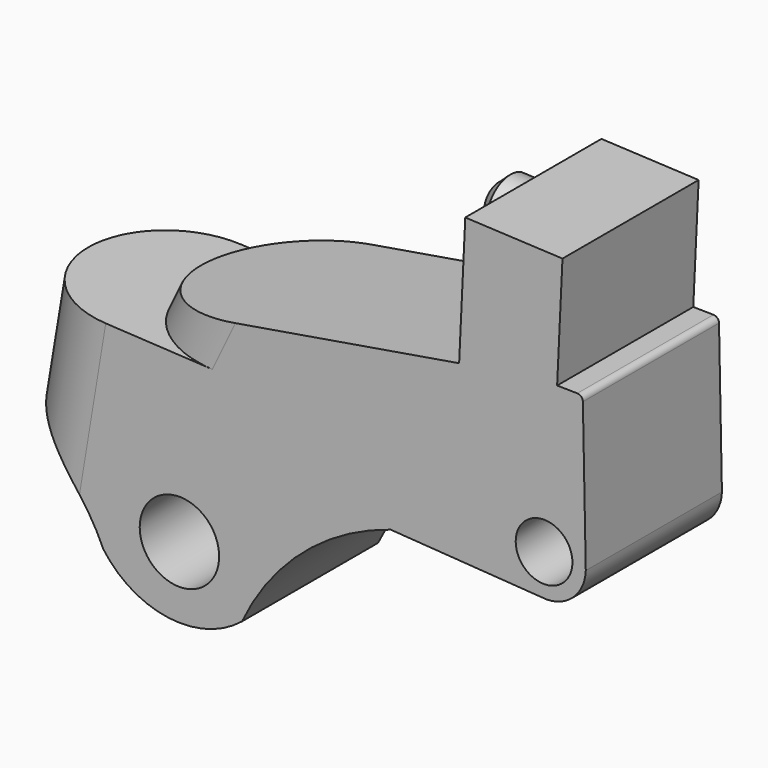
from build123d import *

# Parameters (mm, degrees)
F1_DEPTH = 3.81
F2_D     = 1.778
F3_D     = 1.27
F4_R     = 1.90499
F5_DEPTH = 2.921
F6_R     = 0.636089801
F7_DEPTH = 0.762
F8_SIZE  = 0.254
F9_R     = 0.127


# Not quite as in the source:
# - a fillet or chamfer is up to 0.001 mm smaller than in the source, because OpenCascade refuses the exact size
# - a feature names something its author has since deleted; it is built from what else it names


with BuildPart() as f1:
    # F0 (on Front) → F1 (new body)
    with BuildSketch(Plane.XZ):
        with BuildLine():
            Line((-39.4140869416, 30.484917322), (-39.6941413215, 29.9037330352))
            Line((-39.6941413215, 29.9037330352), (-41.9326054958, 30.025163579))
            Line((-41.9326054958, 30.025163579), (-42.315851897, 27.6998355985))
            ThreePointArc((-42.315851897, 27.6998355985), (-40.9839410359, 26.7856748681), (-40.0724932551, 25.4519060254))
            ThreePointArc((-40.0724932551, 25.4519060254), (-38.6103077884, 24.5752589314), (-36.9695164263, 25.0381845981))
            ThreePointArc((-36.9695164263, 25.0381845981), (-35.6119860231, 26.8367061404), (-33.6415685093, 27.929877378))
            Line((-33.6415685093, 27.929877378), (-30.2701074994, 27.6978733483))
            ThreePointArc((-30.2701074994, 27.6978733483), (-29.5830798604, 27.8997588647), (-29.2723267028, 28.5448923498))
            Line((-29.2723267028, 28.5448923498), (-29.339633882, 31.9740138948))
            Line((-29.339633882, 31.9740138948), (-29.925275594, 31.9827347994))
            Line((-29.925275594, 31.9827347994), (-29.9314986914, 31.6059216857))
            Line((-29.9314986914, 31.6059216857), (-32.1076634707, 31.7085161805))
            Line((-32.1076634707, 31.7085161805), (-39.4140869416, 30.484917322))
        make_face()
    extrude(amount=F1_DEPTH)

    # F2 (through all)
    with Locations(Plane(origin=(0, 0, 0), x_dir=(1, 0, 0), z_dir=(0, 1, 0))):
        with Locations((-38.3695736527, -26.1525325477)):
            Hole(F2_D / 2)

    # F3 (through all)
    with Locations(Plane(origin=(0, 0, 0), x_dir=(1, 0, 0), z_dir=(0, 1, 0))):
        with Locations((-30.2061401308, -28.6094471812)):
            Hole(F3_D / 2)

    # F4 (radius 1.905 in the source; OpenCascade refuses exactly that, so slightly less here)
    f4_edges = [f1.edges().sort_by_distance(p)[0] for p in [
        (-42.124229, -3.81, 28.8625),
        (-42.124229, 0, 28.8625),
        (-39.554114, -3.81, 30.194325),
        (-39.554114, 0, 30.194325),
    ]]
    fillet(f4_edges, radius=F4_R)

    # F5 (add): a face of the model
    f5_faces = [f1.faces().sort_by_distance(p)[0] for p in [
        (-31.0195810811, -1.905, 31.6572189331),
    ]]
    extrude(f5_faces, amount=F5_DEPTH)

    # F6 (on face) → F7 (join)
    with BuildSketch(Plane(origin=(-33.5280299441, 0, 1.5806667432), x_dir=(0, -1, 0), z_dir=(-0.9988905408, 0, 0.0470923302))):
        with Locations((1.905, 32.3275662959)):
            Circle(F6_R)
    extrude(amount=F7_DEPTH)

    # F8
    f8_edges = [f1.edges().sort_by_distance(p)[0] for p in [
        (-32.766804, -1.26891, 33.908251),
    ]]
    chamfer(f8_edges, length=F8_SIZE)

    # F9
    f9_edges = [f1.edges().sort_by_distance(p)[0] for p in [
        (-29.339634, -1.905, 31.974014),
    ]]
    fillet(f9_edges, radius=F9_R)


solid = f1.part
